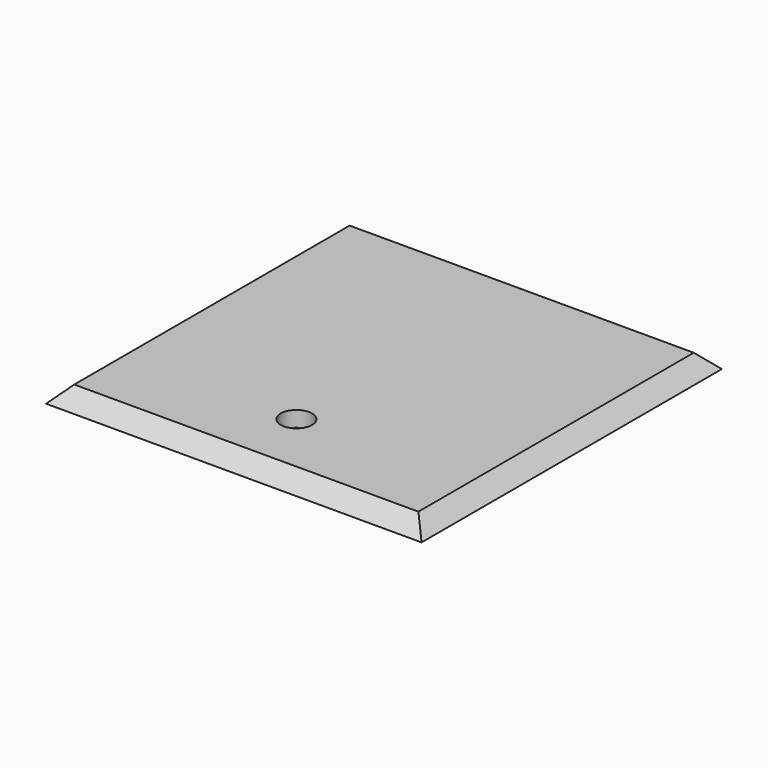
from build123d import *

# Parameters (mm, degrees)
F0_W     = 76.2
F0_H     = 76.2
F0_R     = 3.175
F1_DEPTH = 3.175
F2_SIZE  = 3.17499


# Not quite as in the source:
# - a fillet or chamfer is up to 0.001 mm smaller than in the source, because OpenCascade refuses the exact size


with BuildPart() as f1:
    # F0 (on Top) → F1 (new body)
    with BuildSketch(Plane.XY):
        with Locations((38.1, 38.1)):
            Rectangle(F0_W, F0_H)
        with Locations((38.1, 15.875)):
            Circle(F0_R, mode=Mode.SUBTRACT)
    extrude(amount=F1_DEPTH)

    # F2 (size 3.175 in the source; OpenCascade refuses exactly that, so slightly less here)
    f2_edges = [f1.edges().sort_by_distance(p)[0] for p in [
        (38.1, 76.2, 3.175),
        (76.2, 38.1, 3.175),
        (38.1, 0, 3.175),
        (0, 38.1, 3.175),
    ]]
    chamfer(f2_edges, length=F2_SIZE)


solid = f1.part
